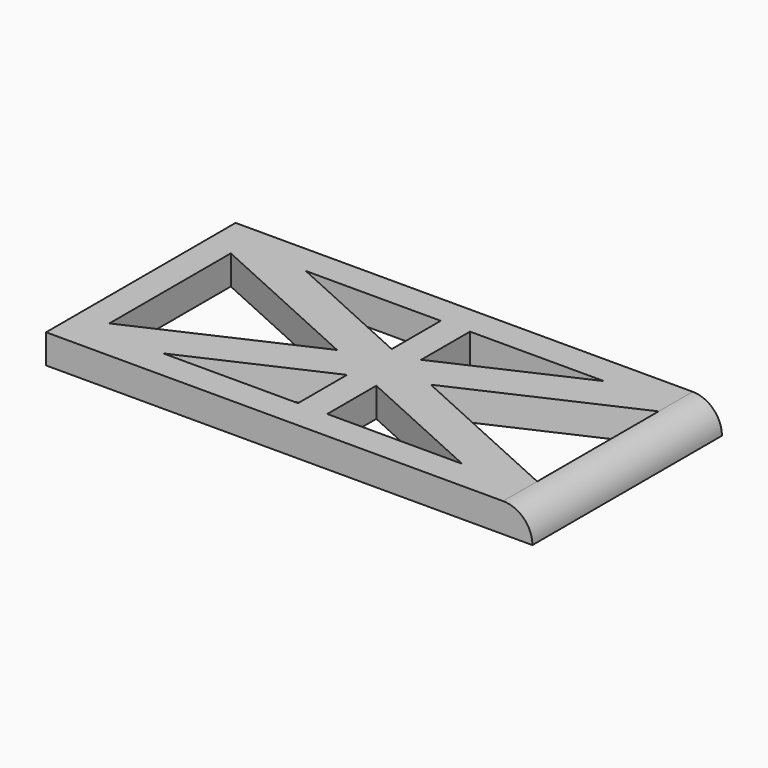
from build123d import *

# Parameters (mm, degrees)
F1_DEPTH = 1
F2_R     = 0.99999


# Not quite as in the source:
# - a fillet or chamfer is up to 0.001 mm smaller than in the source, because OpenCascade refuses the exact size


with BuildPart() as f1:
    # F0 (on Top) → F1 (new body)
    with BuildSketch(Plane.XY):
        Polygon((-7.3084038651, 2.5000789639), (-8.3084038651, 2.9543336025), (-8.3084038651, -3.1456663975), (-7.3084038651, -2.6904001687), align=None)
        Polygon((-7.3084038651, 2.9543336025), (-8.3084038651, 2.9543336025), (-7.3084038651, 2.5000789639), align=None)
        Polygon((-7.3084038651, 3.9543336025), (-8.3084038651, 3.9543336025), (-8.3084038651, 2.9543336025), (-7.3084038651, 2.9543336025), (-5.1069954144, 2.9543336025), align=None)
        Polygon((-7.3084038651, -2.6904001687), (-8.3084038651, -3.1456663975), (-7.3084038651, -3.1456663975), align=None)
        Polygon((-7.3084038651, -3.1456663975), (-8.3084038651, -3.1456663975), (-8.3084038651, -4.1456663975), (-7.3017124087, -4.1456663975), (-5.1012464166, -3.1456663975), align=None)
        Polygon((-0.4934038651, -3.1456663975), (-5.1012464166, -3.1456663975), (-7.3017124087, -4.1456663975), (7.3215961349, -4.1456663975), (5.1201876842, -3.1456663975), (0.5065961349, -3.1456663975), align=None)
        Polygon((-7.3084038651, -2.6904001687), (-7.3084038651, -3.1456663975), (-5.1012464166, -3.1456663975), (-0.4934038651, -1.0516360566), (-0.4934038651, -0.5956663975), (-1.6015758867, -0.0922741165), align=None)
        Polygon((-0.0026520019, 0.6356619308), (-0.4934038651, 0.4122391807), (-0.4934038651, -0.5956663975), (0.0083764092, -0.8236024146), (0.5065961349, -0.597186861), (0.5065961349, 0.4043336025), align=None)
        Polygon((0.0083764092, -0.8236024146), (-0.4934038651, -0.5956663975), (-0.4934038651, -1.0516360566), align=None)
        Polygon((0.5065961349, -0.597186861), (0.0083764092, -0.8236024146), (0.5065961349, -1.0499210361), align=None)
        Polygon((1.6087379174, -0.0963194146), (0.5065961349, 0.4043336025), (0.5065961349, -0.597186861), align=None)
        Polygon((-0.0026520019, 0.6356619308), (-0.4934038651, 0.858588241), (-0.4934038651, 0.4122391807), align=None)
        Polygon((0.5065961349, 0.4043336025), (0.5065961349, 0.8675054096), (-0.0026520019, 0.6356619308), align=None)
        Polygon((0.5065961349, 2.9543336025), (-0.4934038651, 2.9543336025), (-0.4934038651, 0.858588241), (-0.0026520019, 0.6356619308), (0.5065961349, 0.8675054096), align=None)
        Polygon((-0.4934038651, -1.0516360566), (-0.4934038651, -3.1456663975), (0.5065961349, -3.1456663975), (0.5065961349, -1.0499210361), (0.0083764092, -0.8236024146), align=None)
        Polygon((7.3215961349, 2.9543336025), (5.0903496856, 2.9543336025), (0.5065961349, 0.8675054096), (0.5065961349, 0.4043336025), (1.6087379174, -0.0963194146), (7.3215961349, 2.4998844069), align=None)
        Polygon((8.3215961349, 3.9543336025), (7.2868666612, 3.9543336025), (5.0903496856, 2.9543336025), (7.3215961349, 2.9543336025), (8.3215961349, 2.9543336025), align=None)
        Polygon((7.3215961349, 2.4998844069), (8.3215961349, 2.9543336025), (7.3215961349, 2.9543336025), align=None)
        Polygon((8.3215961349, -3.1456663975), (8.3215961349, 2.9543336025), (7.3215961349, 2.4998844069), (7.3215961349, -2.691411759), align=None)
        Polygon((7.3215961349, -3.1456663975), (8.3215961349, -3.1456663975), (7.3215961349, -2.691411759), align=None)
        Polygon((8.3215961349, -4.1456663975), (8.3215961349, -3.1456663975), (7.3215961349, -3.1456663975), (5.1201876842, -3.1456663975), (7.3215961349, -4.1456663975), align=None)
        Polygon((-0.4934038651, 0.858588241), (-5.1069954144, 2.9543336025), (-7.3084038651, 2.9543336025), (-7.3084038651, 2.5000789639), (-1.6015758867, -0.0922741165), (-0.4934038651, 0.4122391807), align=None)
        Polygon((-0.4934038651, 0.4122391807), (-1.6015758867, -0.0922741165), (-0.4934038651, -0.5956663975), align=None)
        Polygon((5.1201876842, -3.1456663975), (7.3215961349, -3.1456663975), (7.3215961349, -2.691411759), (1.6087379174, -0.0963194146), (0.5065961349, -0.597186861), (0.5065961349, -1.0499210361), align=None)
        Polygon((7.2868666612, 3.9543336025), (-7.3084038651, 3.9543336025), (-5.1069954144, 2.9543336025), (-0.4934038651, 2.9543336025), (0.5065961349, 2.9543336025), (5.0903496856, 2.9543336025), align=None)
    extrude(amount=F1_DEPTH)

    # F2 (radius 1 in the source; OpenCascade refuses exactly that, so slightly less here)
    f2_edges = [f1.edges().sort_by_distance(p)[0] for p in [
        (8.321596, -0.095666, 1),
    ]]
    fillet(f2_edges, radius=F2_R)


solid = f1.part
